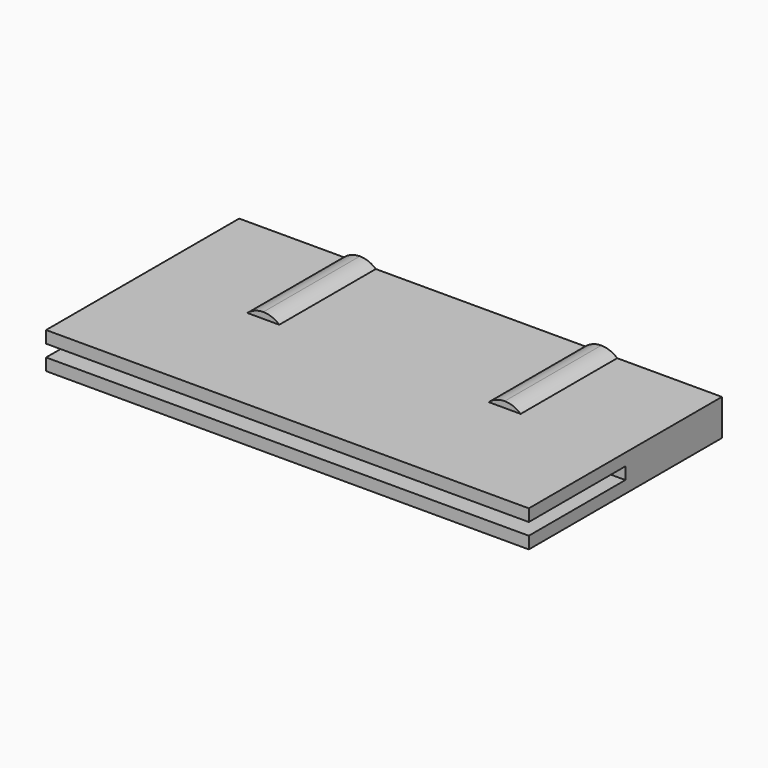
from build123d import *

# Parameters (mm, degrees)
F0_W     = 40
F0_H     = 20
F1_DEPTH = 3
F2_W     = 40
F2_H     = 1
F3_DEPTH = 10
F5_DEPTH = 10
F6_DEPTH = 8


with BuildPart() as f1:
    # F0 (on Top) → F1 (new body)
    with BuildSketch(Plane.XY):
        Rectangle(F0_W, F0_H)
    extrude(amount=F1_DEPTH)

    # F2 (on face) → F3 (cut)
    with BuildSketch(Plane.XZ.offset(10)):
        with Locations((0, 1.5)):
            Rectangle(F2_W, F2_H)
    extrude(amount=-F3_DEPTH, mode=Mode.SUBTRACT)

    # F4 (on face) → F5 (join)
    with BuildSketch(Plane(origin=(0, 10, 0), x_dir=(-1, 0, 0), z_dir=(0, 1, 0))):
        with BuildLine():
            ThreePointArc((10, 3.5), (9.2928932188, 3.3708286934), (8.6771243445, 3))
            Line((8.6771243445, 3), (10, 3))
            Line((10, 3), (10, 3.5))
        make_face()
        with BuildLine():
            Line((-10, 3), (-8.6771243445, 3))
            ThreePointArc((-8.6771243445, 3), (-9.2928932188, 3.3708286934), (-10, 3.5))
            Line((-10, 3.5), (-10, 3))
        make_face()
        with BuildLine():
            ThreePointArc((11.3228756555, 3), (10.7071067812, 3.3708286934), (10, 3.5))
            Line((10, 3.5), (10, 3))
            Line((10, 3), (11.3228756555, 3))
        make_face()
        with BuildLine():
            Line((-10, 3), (-10, 3.5))
            ThreePointArc((-10, 3.5), (-10.7071067812, 3.3708286934), (-11.3228756555, 3))
            Line((-11.3228756555, 3), (-10, 3))
        make_face()
        with BuildLine():
            ThreePointArc((-10, -0.5), (-9.2928932188, -0.3708286934), (-8.6771243445, 0))
            Line((-8.6771243445, 0), (-10, 0))
            Line((-10, 0), (-10, -0.5))
        make_face()
        with BuildLine():
            Line((10, 0), (8.6771243445, 0))
            ThreePointArc((8.6771243445, 0), (9.2928932188, -0.3708286934), (10, -0.5))
            Line((10, -0.5), (10, 0))
        make_face()
        with BuildLine():
            ThreePointArc((-11.3228756555, 0), (-10.7071067812, -0.3708286934), (-10, -0.5))
            Line((-10, -0.5), (-10, 0))
            Line((-10, 0), (-11.3228756555, 0))
        make_face()
        with BuildLine():
            Line((10, 0), (10, -0.5))
            ThreePointArc((10, -0.5), (10.7071067812, -0.3708286934), (11.3228756555, 0))
            Line((11.3228756555, 0), (10, 0))
        make_face()
    extrude(amount=-F5_DEPTH)

    # F4 (on face) → F6 (cut)
    with BuildSketch(Plane(origin=(0, 10, 0), x_dir=(-1, 0, 0), z_dir=(0, 1, 0))):
        with BuildLine():
            ThreePointArc((-10, 2), (-10.5, 1.5), (-10, 1))
            Line((-10, 1), (-10, 2))
        make_face()
        with BuildLine():
            Line((-10, 2), (-10, 1))
            ThreePointArc((-10, 1), (-9.6464466094, 1.1464466094), (-9.5, 1.5))
            ThreePointArc((-9.5, 1.5), (-9.6464466094, 1.8535533906), (-10, 2))
        make_face()
        with BuildLine():
            Line((10, 2), (10, 1))
            ThreePointArc((10, 1), (10.3535533906, 1.1464466094), (10.5, 1.5))
            ThreePointArc((10.5, 1.5), (10.3535533906, 1.8535533906), (10, 2))
        make_face()
        with BuildLine():
            ThreePointArc((10, 2), (9.5, 1.5), (10, 1))
            Line((10, 1), (10, 2))
        make_face()
    extrude(amount=-F6_DEPTH, mode=Mode.SUBTRACT)


solid = f1.part
